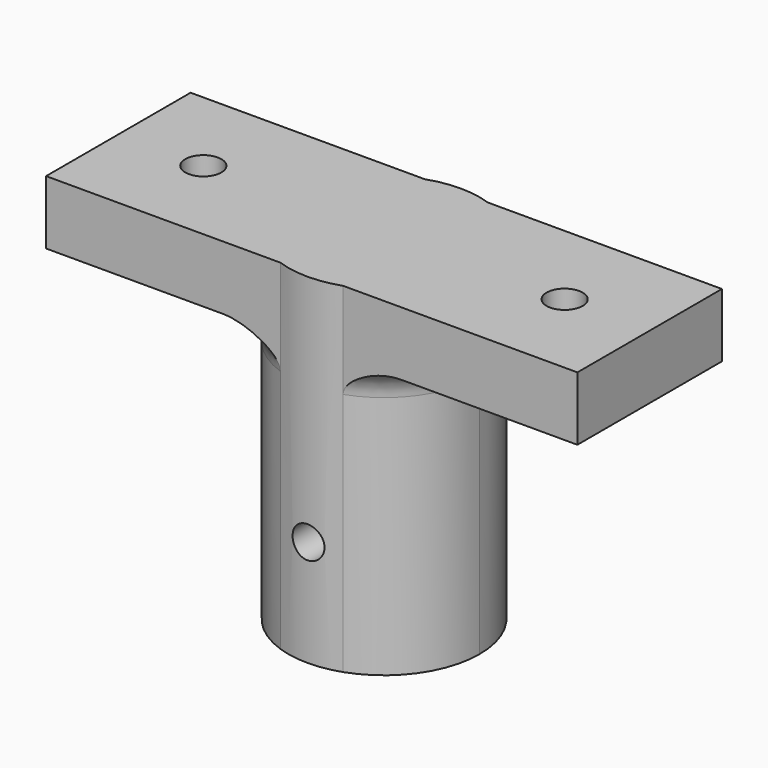
from build123d import *

# Parameters (mm, degrees)
F1_W         = 50
F1_H         = 17
F1_R         = 1.7
F2_DEPTH     = 6
F4_DEPTH     = 32
F5_T4_ANGLE  = 237.2117204573
F5_T10_ANGLE = 237.2117204573
F6_R         = 6
F7_DEPTH     = 25
F8_R         = 1.5
F9_DEPTH     = 15.2


# Not quite as in the source:
# - a fillet or chamfer that OpenCascade refuses, or shapes differently, is made with other operations: its cross-section is extruded or revolved along the edge and cut away or added


with BuildPart() as f2:
    # F1 (on offset) → F2 (new body)
    with BuildSketch(Plane.XY.offset(70)):
        Rectangle(F1_W, F1_H)
        with Locations((-17, 0)):
            Circle(F1_R, mode=Mode.SUBTRACT)
        with Locations((17, 0)):
            Circle(F1_R, mode=Mode.SUBTRACT)
    extrude(amount=-F2_DEPTH)

    # F3 (on face) → F4 (join)
    with BuildSketch(Plane.XY.offset(70)):
        with BuildLine():
            ThreePointArc((2.9580398915, -8.5), (7.3356103708, -5.2142900272), (9, 0))
            ThreePointArc((9, 0), (7.3356103708, 5.2142900272), (2.9580398915, 8.5))
            Line((2.9580398915, 8.5), (-2.9580398916, 8.5))
            ThreePointArc((-2.9580398916, 8.5), (-9, 0), (-2.9580398916, -8.5))
            Line((-2.9580398916, -8.5), (2.9580398915, -8.5))
        make_face()
        with BuildLine():
            ThreePointArc((-2.9580398916, -8.5), (0, -9), (2.9580398915, -8.5))
            Line((2.9580398915, -8.5), (-2.9580398916, -8.5))
        make_face()
        with BuildLine():
            Line((-2.9580398916, 8.5), (2.9580398915, 8.5))
            ThreePointArc((2.9580398915, 8.5), (0, 9), (-2.9580398916, 8.5))
        make_face()
    extrude(amount=-F4_DEPTH)

    # F5: fillet of radius 3 on 2 edges, made by hand


with BuildPart() as f5_tool2:
    # F5_s3 → F5_t4 (revolve)
    with BuildSketch(Plane(origin=(0, 0, 0), x_dir=(0, 0, 1), z_dir=(-0.8779340101, 0.4787816558, 0))):
        with BuildLine():
            ThreePointArc((61, -9), (63.1213203436, -9.8786796564), (64, -12))
            Line((64, -12), (64, -9))
            Line((64, -9), (61, -9))
        make_face()
    revolve(axis=Axis((0, 0, 64), (0, 0, 1)), revolution_arc=F5_T4_ANGLE)

    split(bisect_by=Plane.XZ.offset(-8.5), keep=Keep.TOP)

    split(bisect_by=Plane.XZ.offset(8.5), keep=Keep.BOTTOM)


with BuildPart() as f2_1:
    add(f2.part)

    # F5_t1: union F5_tool2
    add(f5_tool2.part)


with BuildPart() as f5_tool8:
    # F5_s9 → F5_t10 (revolve)
    with BuildSketch(Plane(origin=(0, 0, 0), x_dir=(0, 0, 1), z_dir=(0.8779340101, -0.4787816558, 0))):
        with BuildLine():
            ThreePointArc((61, -9), (63.1213203436, -9.8786796564), (64, -12))
            Line((64, -12), (64, -9))
            Line((64, -9), (61, -9))
        make_face()
    revolve(axis=Axis((0, 0, 64), (0, 0, 1)), revolution_arc=F5_T10_ANGLE)

    split(bisect_by=Plane.XZ.offset(-8.5), keep=Keep.TOP)

    split(bisect_by=Plane.XZ.offset(8.5), keep=Keep.BOTTOM)


with BuildPart() as f2_2:
    add(f2_1.part)

    # F5_t7: union F5_tool8
    add(f5_tool8.part)

    # F6 (on face) → F7 (cut)
    with BuildSketch(Plane(origin=(0, 0, 38), x_dir=(1, 0, 0), z_dir=(0, 0, -1))):
        Circle(F6_R)
    extrude(amount=-F7_DEPTH, mode=Mode.SUBTRACT)

    # F8 (on Front) → F9 (cut, symmetric)
    with BuildSketch(Plane.XZ):
        with Locations((0, 48)):
            Circle(F8_R)
    extrude(amount=F9_DEPTH, both=True, mode=Mode.SUBTRACT)


solid = f2_2.part
